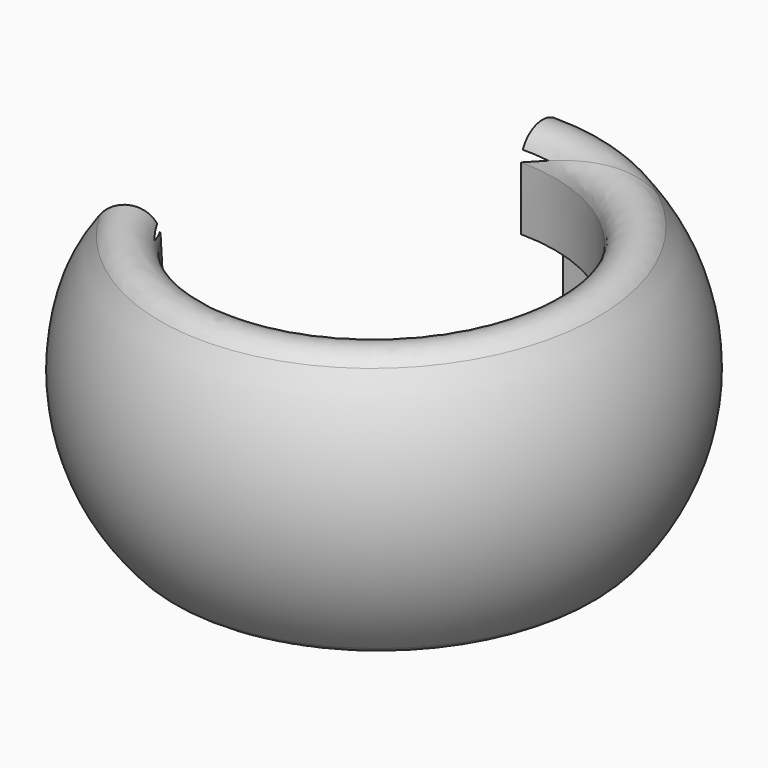
from build123d import *

# Parameters (mm, degrees)
F2_ANGLE    = 240
F3_W        = 7.112
F3_H        = 7.112
F4_DEPTH    = 5.55625
F5_W        = 7.112
F5_H        = 7.112
F6_DEPTH    = 5.55625
F7_T4_ANGLE = 349.948380696
F7_T9_ANGLE = 349.948380696
F8_T4_ANGLE = 343.9133898586
F8_T9_ANGLE = 343.9133898586
F11_DEPTH   = 6.35
F13_DEPTH   = 6.35


# Not quite as in the source:
# - a fillet or chamfer that OpenCascade refuses, or shapes differently, is made with other operations: its cross-section is extruded or revolved along the edge and cut away or added


with BuildPart() as f2:
    # F0 (on Right) → F2 (revolve)
    with BuildSketch(Plane.YZ):
        with BuildLine():
            Line((0, -25.9387402122), (0, -47.9325240122))
            ThreePointArc((0, -47.9325240122), (17.5731218804, -15.7507240122), (0, 16.4310759878))
            Line((0, 16.4310759878), (0, -6.8887402122))
            Line((0, -6.8887402122), (9.8796226174, -6.8887402122))
            Line((9.8796226174, -6.8887402122), (9.8796226174, -25.9387402122))
            Line((9.8796226174, -25.9387402122), (0, -25.9387402122))
        make_face()
    revolve(axis=Axis((0, -32.9686308407, -2.2695437855), (0, 0.0285596631, -0.9995920896)), revolution_arc=F2_ANGLE)

    # F3 (on Right) → F4 (cut)
    with BuildSketch(Plane.YZ):
        with Locations((3.556, 3.556)):
            Rectangle(F3_W, F3_H)
    extrude(amount=F4_DEPTH, mode=Mode.SUBTRACT)

    # F5 (on Right) → F6 (cut)
    with BuildSketch(Plane.YZ):
        with Locations((3.556, -33.1353539076)):
            Rectangle(F5_W, F5_H)
    extrude(amount=F6_DEPTH, mode=Mode.SUBTRACT)

    # F7: fillet of radius 5.08 on 1 edges, made by hand


with BuildPart() as f7_tool2:
    # F7_s3 → F7_t4 (revolve)
    with BuildSketch(Plane(origin=(-15.519406183, -22.1337407382, -0.6323901361), x_dir=(0.8187835052, -0.5741024052, 0), z_dir=(-0.5739453762, -0.8185595508, -0.0233873249))):
        with BuildLine():
            ThreePointArc((-13.6205038164, -36.4192771202), (-16.9439528127, -41.2478681872), (-22.6057068813, -39.7295975294))
            ThreePointArc((-22.6057068813, -39.7295975294), (-18.3618922347, -44.077312283), (-13.4832691044, -47.6983097543))
            Line((-13.4832691044, -47.6983097543), (-13.6205038164, -36.4192771202))
        make_face()
    revolve(axis=Axis((0, -31.638152468, -48.8364677143), (0, 0.0285596631, -0.9995920896)), revolution_arc=F7_T4_ANGLE)

    split(bisect_by=Plane.XZ, keep=Keep.TOP)


with BuildPart() as f2_1:
    add(f2.part)

    # F7_t1: cut F7_tool2
    add(f7_tool2.part, mode=Mode.SUBTRACT)


with BuildPart() as f7_tool7:
    # F7_s8 → F7_t9 (revolve)
    with BuildSketch(Plane(origin=(-15.519406183, -22.1337407382, -0.6323901361), x_dir=(0.8187835052, -0.5741024052, 0), z_dir=(-0.5739453762, -0.8185595508, -0.0233873249))):
        with BuildLine():
            ThreePointArc((-13.6205038164, -36.4192771202), (-16.9439528127, -41.2478681872), (-22.6057068813, -39.7295975294))
            ThreePointArc((-22.6057068813, -39.7295975294), (-18.3618922347, -44.077312283), (-13.4832691044, -47.6983097543))
            Line((-13.4832691044, -47.6983097543), (-13.6205038164, -36.4192771202))
        make_face()
    revolve(axis=Axis((0, -31.638152468, -48.8364677143), (0, 0.0285596631, -0.9995920896)), revolution_arc=F7_T9_ANGLE)

    split(bisect_by=Plane.XZ, keep=Keep.BOTTOM)


with BuildPart() as f2_2:
    add(f2_1.part)

    # F7_t6: cut F7_tool7
    add(f7_tool7.part, mode=Mode.SUBTRACT)

    # F8: fillet of radius 5.08 on 1 edges, made by hand


with BuildPart() as f8_tool2:
    # F8_s3 → F8_t4 (revolve)
    with BuildSketch(Plane(origin=(-16.0256017919, -20.4715562588, -0.5848993354), x_dir=(0.7874231543, -0.6164128292, 0), z_dir=(-0.6162568906, -0.7872239539, -0.0224920256))):
        with BuildLine():
            ThreePointArc((-12.7256800931, 5.3739698626), (-16.1598904571, 10.124422904), (-21.7850242933, 8.4756432802))
            ThreePointArc((-21.7850242933, 8.4756432802), (-17.6428750877, 12.9203239541), (-12.8492834764, 16.6531601142))
            Line((-12.8492834764, 16.6531601142), (-12.7256800931, 5.3739698626))
        make_face()
    revolve(axis=Axis((0, -33.4756053748, 15.4746338351), (0, 0.0285596631, -0.9995920896)), revolution_arc=F8_T4_ANGLE)

    split(bisect_by=Plane.XZ, keep=Keep.TOP)


with BuildPart() as f2_3:
    add(f2_2.part)

    # F8_t1: cut F8_tool2
    add(f8_tool2.part, mode=Mode.SUBTRACT)


with BuildPart() as f8_tool7:
    # F8_s8 → F8_t9 (revolve)
    with BuildSketch(Plane(origin=(-16.0256017919, -20.4715562588, -0.5848993354), x_dir=(0.7874231543, -0.6164128292, 0), z_dir=(-0.6162568906, -0.7872239539, -0.0224920256))):
        with BuildLine():
            ThreePointArc((-12.7256800931, 5.3739698626), (-16.1598904571, 10.124422904), (-21.7850242933, 8.4756432802))
            ThreePointArc((-21.7850242933, 8.4756432802), (-17.6428750877, 12.9203239541), (-12.8492834764, 16.6531601142))
            Line((-12.8492834764, 16.6531601142), (-12.7256800931, 5.3739698626))
        make_face()
    revolve(axis=Axis((0, -33.4756053748, 15.4746338351), (0, 0.0285596631, -0.9995920896)), revolution_arc=F8_T9_ANGLE)

    split(bisect_by=Plane.XZ, keep=Keep.BOTTOM)


with BuildPart() as f2_4:
    add(f2_3.part)

    # F8_t6: cut F8_tool7
    add(f8_tool7.part, mode=Mode.SUBTRACT)

    # F10 (on offset) → F11 (cut)
    with BuildSketch(Plane(origin=(14.2980794165, -24.7548980996, -0.7072800555), x_dir=(-0.8660254038, -0.4997960448, -0.0142798315), z_dir=(-0.5, 0.865672143, 0.0247333937))):
        Polygon((49.7467838827, 7.2109422366), (49.8148426414, 0), (56.9025047774, 0), (56.9025047774, 7.2109422366), align=None)
    extrude(amount=-F11_DEPTH, mode=Mode.SUBTRACT)

    # F12 (on offset) → F13 (cut)
    with BuildSketch(Plane(origin=(14.2980794165, -24.7548980996, -0.7072800555), x_dir=(-0.8660254038, -0.4997960448, -0.0142798315), z_dir=(-0.5, 0.865672143, 0.0247333937))):
        Polygon((55.8907425518, -30.6380988543), (48.7787425518, -30.6380988543), (48.716083169, -37.7500988543), (55.8907425518, -37.7500988543), align=None)
    extrude(amount=-F13_DEPTH, mode=Mode.SUBTRACT)


solid = f2_4.part
